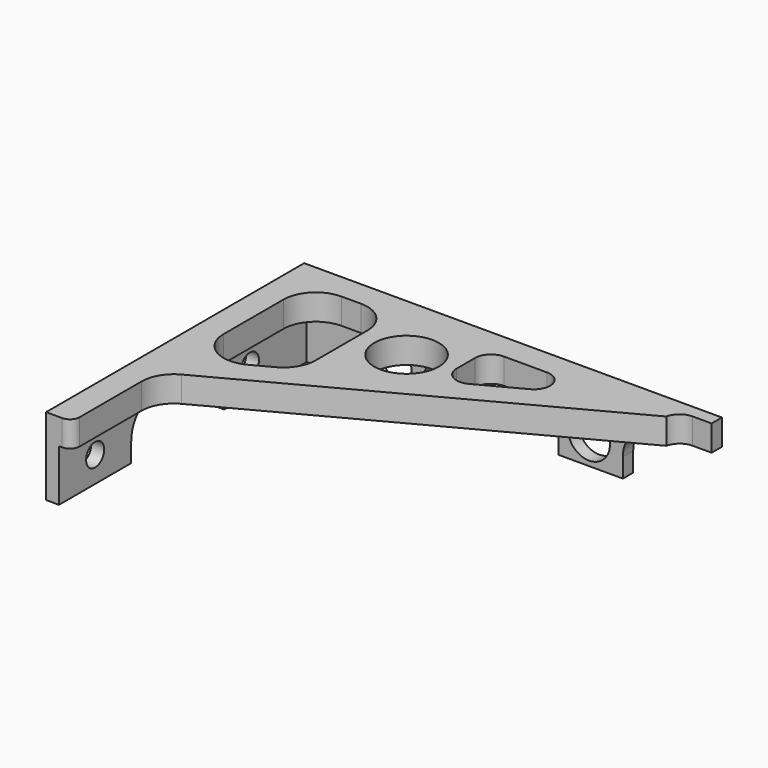
from build123d import *

# Parameters (mm, degrees)
F0_R        = 5
F1_DEPTH    = 4
F2_W        = 10
F2_H        = 2
F2_W_2      = 18
F2_W_3      = 2
F2_H_2      = 14
F3_DEPTH    = 8
F4_R        = 5
F5_T1_DEPTH = 4
F6_R        = 1.5
F8_R        = 3.25
F9_DEPTH    = 2
F7_R        = 1.75
F10_DEPTH   = 2


# Not quite as in the source:
# - a fillet or chamfer that OpenCascade refuses, or shapes differently, is made with other operations: its cross-section is extruded or revolved along the edge and cut away or added


with BuildPart() as f1:
    # F0 (on Top) → F1 (new body)
    with BuildSketch(Plane.XY):
        Polygon((-24.0443362383, -18.3656413368), (31.299512524, 11.1093264446), (31.299512524, 13.1093264446), (36.7056637617, 13.1093264446), (36.7056637617, 15.1093264446), (-28.0443362383, 15.1093264446), (-28.0443362383, -34.8906735554), (-24.0443362383, -34.8906735554), align=None)
        Polygon((-24.0443362383, -13.8337272738), (-24.0443362383, 11.1093264446), (-11.0443362383, 11.1093264446), (3.6275881428, 11.1093264446), (22.7901370984, 11.1093264446), (3.6275881428, 0.9037566169), (-11.0443362383, -6.9102011778), align=None, mode=Mode.SUBTRACT)
        Polygon((3.6275881428, 11.1093264446), (-11.0443362383, 11.1093264446), (-11.0443362383, -6.9102011778), (3.6275881428, 0.9037566169), align=None)
        with Locations((-3.3724118572, 4.1093264446)):
            Circle(F0_R, mode=Mode.SUBTRACT)
    extrude(amount=F1_DEPTH)

    # F2 (on Top) → F3 (join)
    with BuildSketch(Plane.XY):
        with Locations((17.9556637617, 14.1093264446)):
            Rectangle(F2_W, F2_H)
        with Locations((-17.0443362383, 14.1093264446)):
            Rectangle(F2_W_2, F2_H)
        Polygon((-26.0443362383, 15.1093264446), (-28.0443362383, 15.1093264446), (-28.0443362383, -2.8906735554), (-26.0443362383, -2.8906735554), (-26.0443362383, 13.1093264446), align=None)
        with Locations((-27.0443362383, -27.8906735554)):
            Rectangle(F2_W_3, F2_H_2)
    extrude(amount=-F3_DEPTH)

    # F4
    f4_edges = [f1.edges().sort_by_distance(p)[0] for p in [
        (-24.044336, -18.365641, 2),
        (-24.044336, 11.109326, 2),
        (-8.044336, 14.109326, 0),
        (22.955664, 14.109326, 0),
        (-27.044336, -2.890674, 0),
        (12.955664, 14.109326, 0),
        (-27.044336, -20.890674, 0),
        (-11.044336, -6.910201, 2),
        (-24.044336, -13.833727, 2),
        (-11.044336, 11.109326, 2),
    ]]
    fillet(f4_edges, radius=F4_R)

    # F5: fillet of radius 2.5 on 4 edges, made by hand

    # F5_s2 → F5_t1 (join)
    with BuildSketch(Plane.XY):
        with BuildLine():
            ThreePointArc((31.299512524, 11.1093264446), (32.1678634367, 12.5458181177), (33.7490022668, 13.1093264446))
            Line((33.7490022668, 13.1093264446), (31.299512524, 13.1093264446))
            Line((31.299512524, 13.1093264446), (31.299512524, 11.1093264446))
        make_face()
        with BuildLine():
            ThreePointArc((12.7776375713, 11.1093264446), (15.2031718358, 9.2149530062), (13.9528119525, 6.4027532703))
            Line((13.9528119525, 6.4027532703), (22.7901370984, 11.1093264446))
            Line((22.7901370984, 11.1093264446), (12.7776375713, 11.1093264446))
        make_face()
        with BuildLine():
            ThreePointArc((3.6275881428, 5.0676502325), (4.840719065, 2.9242958576), (7.302762524, 2.8610770581))
            Line((7.302762524, 2.8610770581), (3.6275881428, 0.9037566169))
            Line((3.6275881428, 0.9037566169), (3.6275881428, 5.0676502325))
        make_face()
        with BuildLine():
            ThreePointArc((6.1275881428, 11.1093264446), (4.3598211899, 10.3770933976), (3.6275881428, 8.6093264446))
            Line((3.6275881428, 8.6093264446), (3.6275881428, 11.1093264446))
            Line((3.6275881428, 11.1093264446), (6.1275881428, 11.1093264446))
        make_face()
    extrude(amount=F5_T1_DEPTH)

    # F6
    f6_edges = [f1.edges().sort_by_distance(p)[0] for p in [
        (-24.044336, -34.890674, 2),
    ]]
    fillet(f6_edges, radius=F6_R)

    # F8 (on face) → F9 (cut)
    with BuildSketch(Plane(origin=(0, 15.1093264446, 0), x_dir=(-1, 0, 0), z_dir=(0, 1, 0))):
        with Locations((-17.7056637617, -4)):
            Circle(F8_R)
        with Locations((13.0443362383, -4)):
            Circle(F8_R)
    extrude(amount=-F9_DEPTH, mode=Mode.SUBTRACT)

    # F7 (on face) → F10 (cut)
    with BuildSketch(Plane(origin=(-28.0443362383, 0, 0), x_dir=(0, -1, 0), z_dir=(-1, 0, 0))):
        with Locations((27.8906735554, -4)):
            Circle(F7_R)
        with Locations((-2.1093264446, -4)):
            Circle(F7_R)
    extrude(amount=-F10_DEPTH, mode=Mode.SUBTRACT)


solid = f1.part
